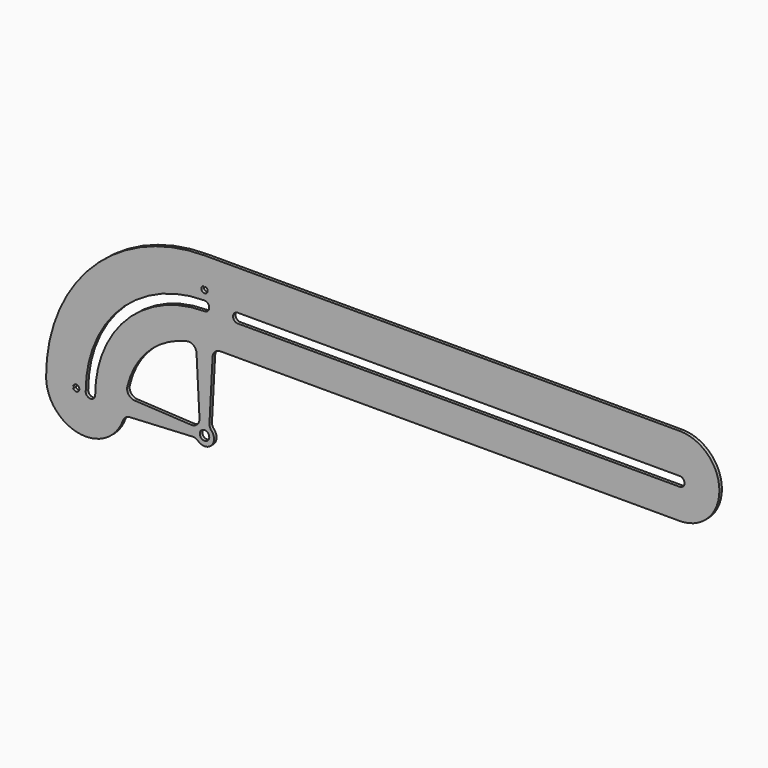
from build123d import *

# Parameters (mm, degrees)
F0_R     = 3
F1_DEPTH = 1
F2_R     = 5
F2_R_2   = 4.99999
F6_DEPTH = 25


# Not quite as in the source:
# - a fillet or chamfer is up to 0.001 mm smaller than in the source, because OpenCascade refuses the exact size
# - a feature of the source that left no trace in its solid (it failed there, or was rolled back) is left out


with BuildPart() as f1:
    # F0 (on Front) → F1 (new body, symmetric)
    with BuildSketch(Plane.XZ):
        with BuildLine():
            ThreePointArc((-70.8333333333, 24.6503324296), (-91.1374306092, 19.0940653956), (-100, 0))
            ThreePointArc((-100, 0), (-77.7052620956, -24.8532001359), (-50.5854754405, -5.3787536225))
            ThreePointArc((-50.5854754405, -5.3787536225), (-50.1467998641, -2.7052620956), (-50, 0))
            ThreePointArc((-50, 0), (-54.1054233512, 13.7264950613), (-65.0733333333, 22.9447442542))
            ThreePointArc((-65.0733333333, 22.9447442542), (-68.0112490695, 11.6391580452), (-69, 0))
            ThreePointArc((-69, 0), (-72, -3), (-75, 0))
            ThreePointArc((-75, 0), (-73.9509972887, 12.5), (-70.8333333333, 24.6503324296))
        make_face()
        with BuildLine():
            ThreePointArc((-50, 0), (-50.1467998641, -2.7052620956), (-50.5854754405, -5.3787536225))
            Line((-50.5854754405, -5.3787536225), (-5.1961524227, -3))
            ThreePointArc((-5.1961524227, -3), (-6, 0), (-5.1961524227, 3))
            Line((-5.1961524227, 3), (-49.7147645476, 5.3331215982))
            ThreePointArc((-49.7147645476, 5.3331215982), (-49.9286402147, 2.6703719425), (-50, 0))
        make_face()
        with BuildLine():
            Line((300, 100), (0, 100))
            ThreePointArc((0, 100), (-70.7106781187, 70.7106781187), (-100, 0))
            ThreePointArc((-100, 0), (-91.1374306092, 19.0940653956), (-70.8333333333, 24.6503324296))
            ThreePointArc((-70.8333333333, 24.6503324296), (-43.4524168935, 61.1300864232), (0, 75))
            ThreePointArc((0, 75), (2.1213203436, 74.1213203436), (3, 72))
            ThreePointArc((3, 72), (2.1213203436, 69.8786796564), (0, 69))
            ThreePointArc((0, 69), (-39.861087833, 56.3213429951), (-65.0733333333, 22.9447442542))
            ThreePointArc((-65.0733333333, 22.9447442542), (-54.1054233512, 13.7264950613), (-50, 0))
            ThreePointArc((-50, 0), (-49.9286402147, 2.6703719425), (-49.7147645476, 5.3331215982))
            ThreePointArc((-49.7147645476, 5.3331215982), (-35.3553390593, 35.3553390593), (-5.3331215982, 49.7147645476))
            ThreePointArc((-5.3331215982, 49.7147645476), (-2.6703719425, 49.9286402147), (0, 50))
            Line((0, 50), (5.3480701549, 50))
            Line((5.3480701549, 50), (300, 50))
            ThreePointArc((300, 50), (284.5889649926, 55.314980315), (275.730677801, 69))
            Line((275.730677801, 69), (21, 69))
            ThreePointArc((21, 69), (18, 72), (21, 75))
            Line((21, 75), (275, 75))
            ThreePointArc((275, 75), (282.3223304703, 92.6776695297), (300, 100))
        make_face()
        with BuildLine():
            Line((3, 5.1961524227), (5.3480701549, 50))
            Line((5.3480701549, 50), (0, 50))
            ThreePointArc((0, 50), (-2.6703719425, 49.9286402147), (-5.3331215982, 49.7147645476))
            Line((-5.3331215982, 49.7147645476), (-3, 5.1961524227))
            ThreePointArc((-3, 5.1961524227), (0, 6), (3, 5.1961524227))
        make_face()
        with BuildLine():
            ThreePointArc((-5.1961524227, 3), (-6, 0), (-5.1961524227, -3))
            ThreePointArc((-5.1961524227, -3), (1.5529142706, -5.7955549577), (6, 0))
            ThreePointArc((6, 0), (5.1961524227, 3), (3, 5.1961524227))
            ThreePointArc((3, 5.1961524227), (0, 6), (-3, 5.1961524227))
            ThreePointArc((-3, 5.1961524227), (-4.2426406871, 4.2426406871), (-5.1961524227, 3))
        make_face()
        Circle(F0_R, mode=Mode.SUBTRACT)
        with BuildLine():
            ThreePointArc((325, 75), (317.6776695297, 92.6776695297), (300, 100))
            ThreePointArc((300, 100), (282.3223304703, 92.6776695297), (275, 75))
            Line((275, 75), (300, 75))
            ThreePointArc((300, 75), (302.1213203436, 74.1213203436), (303, 72))
            ThreePointArc((303, 72), (302.1213203436, 69.8786796564), (300, 69))
            Line((300, 69), (275.730677801, 69))
            ThreePointArc((275.730677801, 69), (284.5889649926, 55.314980315), (300, 50))
            ThreePointArc((300, 50), (317.6776695297, 57.3223304703), (325, 75))
        make_face()
    extrude(amount=F1_DEPTH, both=True)

    # F2 (call 1 of 8: OpenCascade refuses the feature's edges together)
    f2_edges = [f1.edges().sort_by_distance(p)[0] for p in [
        (-49.714765, 0, 5.333122),
    ]]
    fillet(f2_edges, radius=F2_R)

    # F2#2 (call 2 of 8)
    f2_2_edges = [f1.edges().sort_by_distance(p)[0] for p in [
        (5.34807, 0, 50),
    ]]
    fillet(f2_2_edges, radius=F2_R)

    # F2#3 (call 3 of 8)
    f2_3_edges = [f1.edges().sort_by_distance(p)[0] for p in [
        (-5.333122, 0, 49.714765),
    ]]
    fillet(f2_3_edges, radius=F2_R)

    # F2#4 (call 4 of 8)
    f2_4_edges = [f1.edges().sort_by_distance(p)[0] for p in [
        (-5.196152, 0, -3),
    ]]
    fillet(f2_4_edges, radius=F2_R)

    # F2#5 (call 5 of 8)
    f2_5_edges = [f1.edges().sort_by_distance(p)[0] for p in [
        (-50.585475, 0, -5.378754),
    ]]
    fillet(f2_5_edges, radius=F2_R)

    # F2#6 (call 6 of 8)
    f2_6_edges = [f1.edges().sort_by_distance(p)[0] for p in [
        (-5.196152, 0, 3),
    ]]
    fillet(f2_6_edges, radius=F2_R)

    # F2#7 (call 7 of 8) (radius 5 in the source; OpenCascade refuses exactly that, so slightly less here)
    f2_7_edges = [f1.edges().sort_by_distance(p)[0] for p in [
        (-3, 0, 5.196152),
    ]]
    fillet(f2_7_edges, radius=F2_R_2)

    # F2#8 (call 8 of 8)
    f2_8_edges = [f1.edges().sort_by_distance(p)[0] for p in [
        (3, 0, 5.196152),
    ]]
    fillet(f2_8_edges, radius=F2_R)

    # F5 (on face) → F6 (cut)
    with BuildSketch(Plane.XZ.offset(1)):
        with BuildLine():
            Line((-82, 0), (-79, 0))
            ThreePointArc((-79, 0), (-80.6813707911, 1.9744557294), (-82.8984754272, 0.629119267))
            Line((-82.8984754272, 0.629119267), (-82, 0))
        make_face()
        with BuildLine():
            ThreePointArc((-82.8984754272, -0.629119267), (-80.6813707911, -1.9744557294), (-79, 0))
            Line((-79, 0), (-82, 0))
            Line((-82, 0), (-82.8984754272, -0.629119267))
        make_face()
        with BuildLine():
            ThreePointArc((-0.629119267, 82.8984754272), (-1.9744557294, 80.6813707911), (0, 79))
            Line((0, 79), (0, 82))
            Line((0, 82), (-0.629119267, 82.8984754272))
        make_face()
        with BuildLine():
            Line((0, 82), (0, 79))
            ThreePointArc((0, 79), (1.4142135624, 79.5857864376), (2, 81))
            ThreePointArc((2, 81), (1.6214559097, 82.1708461611), (0.629119267, 82.8984754272))
            Line((0.629119267, 82.8984754272), (0, 82))
        make_face()
    extrude(amount=-F6_DEPTH, mode=Mode.SUBTRACT)


solid = f1.part
